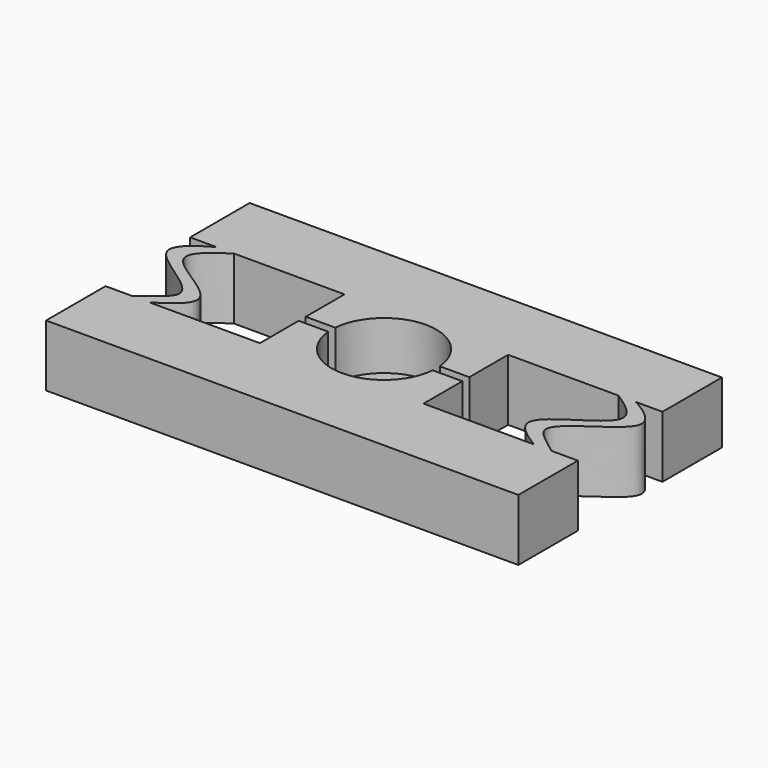
from build123d import *

# Parameters (mm, degrees)
F2_W     = 113.5670877993
F2_H     = 81.1927579343
F2_R     = 31.9732071905
F2_W_2   = 53.6017529666
F2_H_2   = 28.8779456168
F3_DEPTH = 25
F5_DEPTH = 25
F7_DEPTH = 7


with BuildPart() as f1:
    # F0 (on Front) → F1 (revolve)
    with BuildSketch(Plane.XZ):
        Polygon((-5.95, -0.4022617794), (-31.9732071905, -0.4022617794), (-31.9732071905, -7.4022617794), (-4, -7.4022617794), (-4, -5.9022617794), (-5.95, -5.9022617794), align=None)
    revolve(axis=Axis((0, 0, -6.3669939991), (0, 0, 1)))

    # F2 (on face) → F3 (cut)
    with BuildSketch(Plane(origin=(0, 0, -7.4022617794), x_dir=(1, 0, 0), z_dir=(0, 0, -1))):
        with Locations((1.571347937, -4.5206267387)):
            Rectangle(F2_W, F2_H)
        Circle(F2_R, mode=Mode.SUBTRACT)
        Circle(F2_R)
        Rectangle(F2_W_2, F2_H_2, mode=Mode.SUBTRACT)
    extrude(amount=-F3_DEPTH, mode=Mode.SUBTRACT)

    # F4 (on face) → F5 (cut)
    with BuildSketch(Plane(origin=(0, 0, -7.4022617794), x_dir=(1, 0, 0), z_dir=(0, 0, -1))):
        with BuildLine():
            Line((-3.9686269666, 0.5), (-9.2835435644, 0.5))
            Line((-9.2835435644, 0.5), (-9.2835435644, 6))
            Line((-9.2835435644, 6), (-26.8008764833, 6))
            Line((-26.8008764833, 6), (-26.8008764833, -6))
            Line((-26.8008764833, -6), (-9.2835435644, -6))
            Line((-9.2835435644, -6), (-9.2835435644, -0.5))
            Line((-9.2835435644, -0.5), (-3.9686269666, -0.5))
            ThreePointArc((-3.9686269666, -0.5), (-4, 0), (-3.9686269666, 0.5))
        make_face()
        with BuildLine():
            Line((9.2835435644, 0.5), (3.9686269666, 0.5))
            ThreePointArc((3.9686269666, 0.5), (3.9921490369, 0.2504916502), (4, 0))
            ThreePointArc((4, 0), (3.9921490369, -0.2504916502), (3.9686269666, -0.5))
            Line((3.9686269666, -0.5), (9.2835435644, -0.5))
            Line((9.2835435644, -0.5), (9.2835435644, -6))
            Line((9.2835435644, -6), (26.8008764833, -6))
            Line((26.8008764833, -6), (26.8008764833, 6))
            Line((26.8008764833, 6), (9.2835435644, 6))
            Line((9.2835435644, 6), (9.2835435644, 0.5))
        make_face()
    extrude(amount=-F5_DEPTH, mode=Mode.SUBTRACT)

    # F6 (on face) → F7 (join, through all)
    with BuildSketch(Plane(origin=(0, 0, -7.4022617794), x_dir=(1, 0, 0), z_dir=(0, 0, -1))):
        with BuildLine():
            Line((-21.8008764833, 6), (-23.8008764833, 6))
            add(Edge.make_bspline(
                [(-23.8008764833, 6), (-22.2108428095, 4.7094736127), (-19.3347207095, 3.1365293538), (-23.8174722022, -0.0420631575), (-28.2006493816, -2.9682767239), (-25.523675908, -5.0459788725), (-23.8008764833, -6)],
                knots=[0, 0, 0, 0, 0.25, 0.5, 0.75, 1, 1, 1, 1], degree=3))
            Line((-23.8008764833, -6), (-21.8008764833, -6))
            add(Edge.make_bspline(
                [(-21.8008764833, 6), (-20.2684628372, 5.0384721173), (-17.3238246823, 2.9890179574), (-21.7691782562, -0.0192710268), (-26.4047211931, -2.9119338502), (-23.0797043121, -5.1926403316), (-21.8008764833, -6)],
                knots=[0, 0, 0, 0, 0.25, 0.5, 0.75, 1, 1, 1, 1], degree=3))
        make_face()
        with BuildLine():
            add(Edge.make_bspline(
                [(23.8008764833, 6), (22.2108428095, 4.7094736127), (19.3347207095, 3.1365293538), (23.8174722022, -0.0420631575), (28.2006493816, -2.9682767239), (25.523675908, -5.0459788725), (23.8008764833, -6)],
                knots=[0, 0, 0, 0, 0.25, 0.5, 0.75, 1, 1, 1, 1], degree=3))
            Line((23.8008764833, 6), (21.8008764833, 6))
            add(Edge.make_bspline(
                [(21.8008764833, 6), (20.2684628372, 5.0384721173), (17.3238246823, 2.9890179574), (21.7691782562, -0.0192710268), (26.4047211931, -2.9119338502), (23.0797043121, -5.1926403316), (21.8008764833, -6)],
                knots=[0, 0, 0, 0, 0.25, 0.5, 0.75, 1, 1, 1, 1], degree=3))
            Line((21.8008764833, -6), (23.8008764833, -6))
        make_face()
    extrude(amount=-F7_DEPTH)


solid = f1.part
